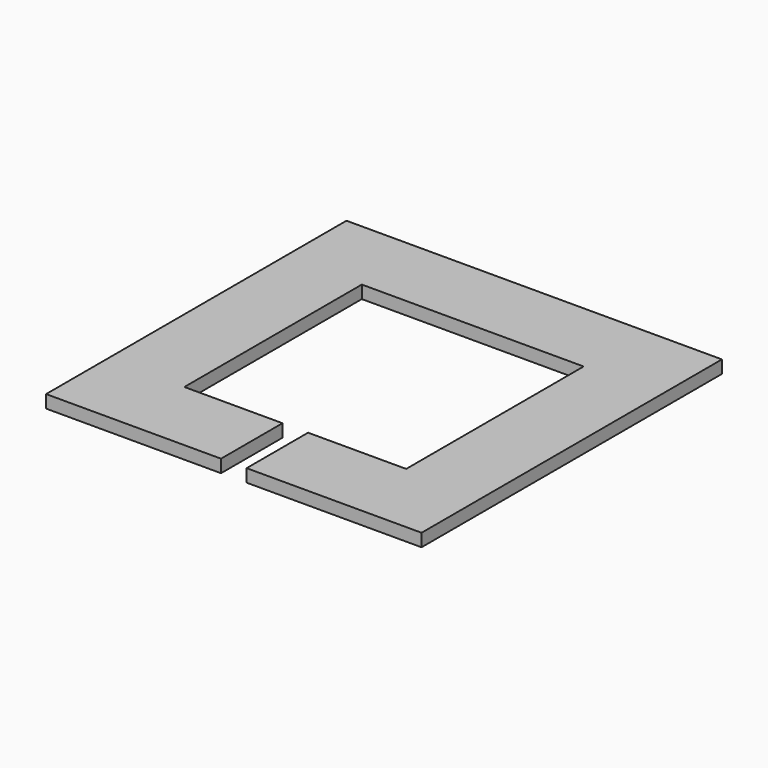
from build123d import *

# Parameters (mm, degrees)
F1_DEPTH = 3.175


# Not quite as in the source:
# - a length typed as a fraction of an inch, garbled in the dataset ("3 / 203.2 mm" for 3/8 in), is restored


with BuildPart() as f1:
    # F0 (on Top) → F1 (new body)
    with BuildSketch(Plane.XY):
        Polygon((46.55, 0), (-46.55, 0), (-46.55, -93.1), (-3.175, -93.1), (-3.175, -74.05), (-27.5, -74.05), (-27.5, -19.05), (27.5, -19.05), (27.5, -74.05), (3.175, -74.05), (3.175, -93.1), (46.55, -93.1), align=None)
    extrude(amount=F1_DEPTH)


solid = f1.part
